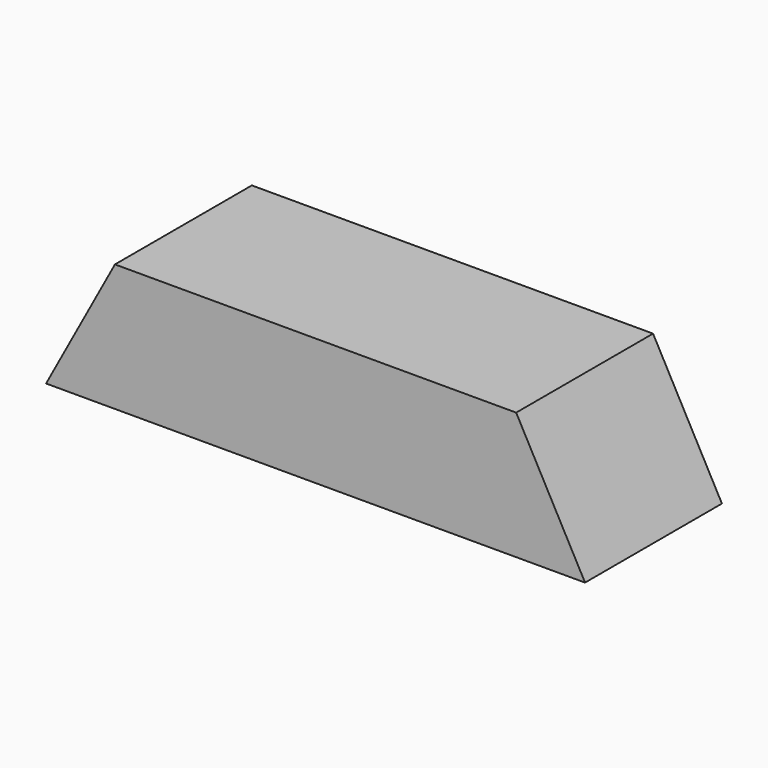
from build123d import *

# Parameters (mm, degrees)
F1_DEPTH = 12.7


# Not quite as in the source:
# - the program builds the solid bodies; features that only make, move or delete a surface that nothing else refers to are left out


with BuildPart() as f1:
    # F0 (on Front) → F1 (new body, symmetric)
    with BuildSketch(Plane.XZ):
        Polygon((-40.0050021708, 0), (0, 0), (40.0050021708, 0), (29.7814980149, 18.891248852), (0, 18.891248852), (-29.7814980149, 18.891248852), align=None)
    extrude(amount=F1_DEPTH, both=True)


solid = f1.part
